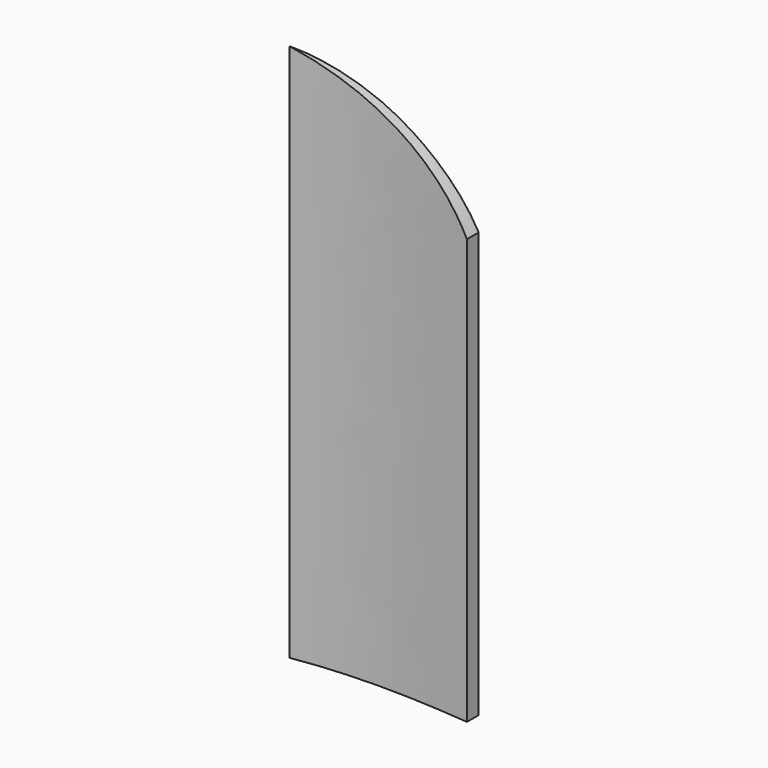
from build123d import *

# Parameters (mm, degrees)
F1_DEPTH = 203.2
F3_DEPTH = 156.21


with BuildPart() as f1:
    # F0 (on Top) → F1 (new body)
    with BuildSketch(Plane.XY):
        with BuildLine():
            add(Edge.make_bspline(
                [(-55.7034760714, 43.3528199792), (-44.8815132724, 48.0532698058), (-28.3737618921, 49.6900983133), (-14.4572808843, 49.5905550092)],
                knots=[0, 0, 0, 0, 30.0627933739, 30.0627933739, 30.0627933739, 30.0627933739], degree=3))
            add(Edge.make_bspline(
                [(-55.7034760714, 43.3528199792), (-32.3167637629, 47.1038674269), (-8.9875221509, 45.8957304569), (10.2285053581, 44.0720804036)],
                knots=[0, 0, 0, 0, 65.9359045648, 65.9359045648, 65.9359045648, 65.9359045648], degree=3))
            Line((10.2285053581, 44.0720804036), (10.2285053581, 46.4467329389))
            add(Edge.make_bspline(
                [(-14.4572808843, 49.5905550092), (-2.7583239734, 49.5068734503), (7.109380778, 48.1960970026), (10.2285053581, 46.4467329389)],
                knots=[30.0627933739, 30.0627933739, 30.0627933739, 30.0627933739, 55.3352256868, 55.3352256868, 55.3352256868, 55.3352256868], degree=3))
        make_face()
        with BuildLine():
            Line((10.2285053581, 49.5905550092), (-14.4572808843, 49.5905550092))
            add(Edge.make_bspline(
                [(-14.4572808843, 49.5905550092), (-2.7583239734, 49.5068734503), (7.109380778, 48.1960970026), (10.2285053581, 46.4467329389)],
                knots=[30.0627933739, 30.0627933739, 30.0627933739, 30.0627933739, 55.3352256868, 55.3352256868, 55.3352256868, 55.3352256868], degree=3))
            Line((10.2285053581, 46.4467329389), (10.2285053581, 49.5905550092))
        make_face()
    extrude(amount=F1_DEPTH)

    # F2 (on Front) → F3 (cut)
    with BuildSketch(Plane.XZ):
        with BuildLine():
            Line((61.6448372602, 207.9568654299), (-86.5255817771, 207.9568654299))
            add(Edge.make_bspline(
                [(-86.5255817771, 207.9568654299), (-24.8807463795, 198.6730098724), (13.3687593043, 174.9063283205), (17.4536593258, 136.285468936)],
                knots=[0, 0, 0, 0, 126.2872584853, 126.2872584853, 126.2872584853, 126.2872584853], degree=3))
            Line((17.4536593258, 136.285468936), (61.6448372602, 207.9568654299))
        make_face()
    extrude(amount=-F3_DEPTH, mode=Mode.SUBTRACT)


solid = f1.part
